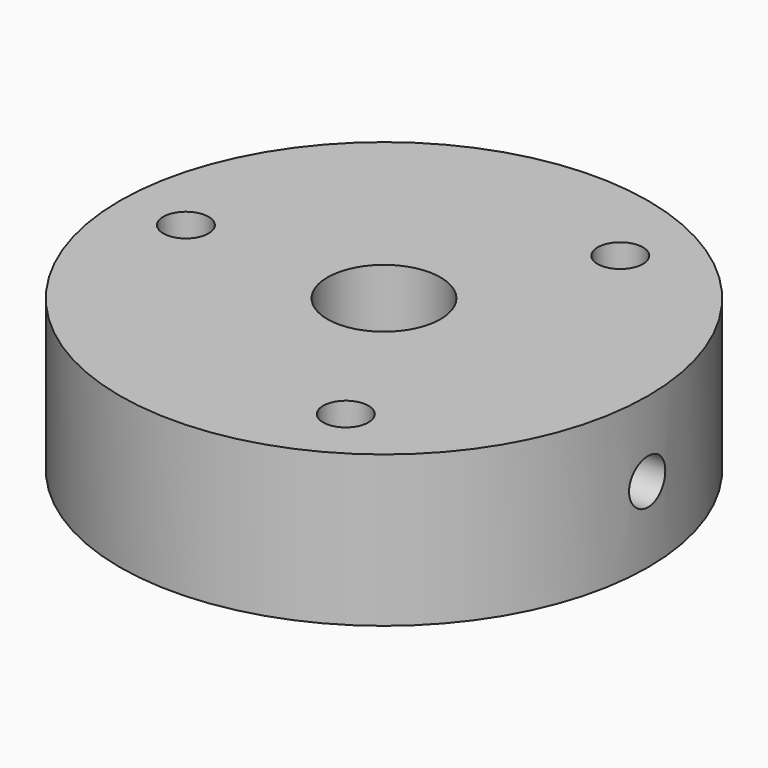
from build123d import *

# Parameters (mm, degrees)
F0_R            = 14
F1_DEPTH        = 8
F3_D            = 6
F4_D            = 2.4
F4_COPIES_COUNT = 3
F6_D            = 2.4
F6_DEPTH        = 14.001


# Not quite as in the source:
# - a pattern or mirror of a feature is missing from the dataset's text; its kind, count and spacing are read off the source's solid


with BuildPart() as f1:
    # F0 (on Top) → F1 (new body)
    with BuildSketch(Plane.XY):
        Circle(F0_R)
    extrude(amount=F1_DEPTH)

    # F3 (through all)
    with Locations(Plane.XY.offset(8)):
        with Locations((0, 0)):
            Hole(F3_D / 2)

    # F4 (through all)
    with Locations(Plane.XY.offset(8)):
        with Locations((-10.5, 0)):
            f4 = Hole(F4_D / 2)

    # F4_copies: F4 ×3 about axis
    f4_copies_axis = Axis((0, 0, 0), (0, 0, 1))
    for i in range(1, F4_COPIES_COUNT):
        add(f4.rotate(f4_copies_axis, i * 360 / F4_COPIES_COUNT), mode=Mode.SUBTRACT)

    # F6 (through all, one way)
    with BuildSketch(Plane(origin=(0, 0, 0), x_dir=(0, 1, 0), z_dir=(-1, 0, 0))):
        with Locations((0, -4)):
            Circle(F6_D / 2)
    extrude(amount=-F6_DEPTH, mode=Mode.SUBTRACT)


solid = f1.part
